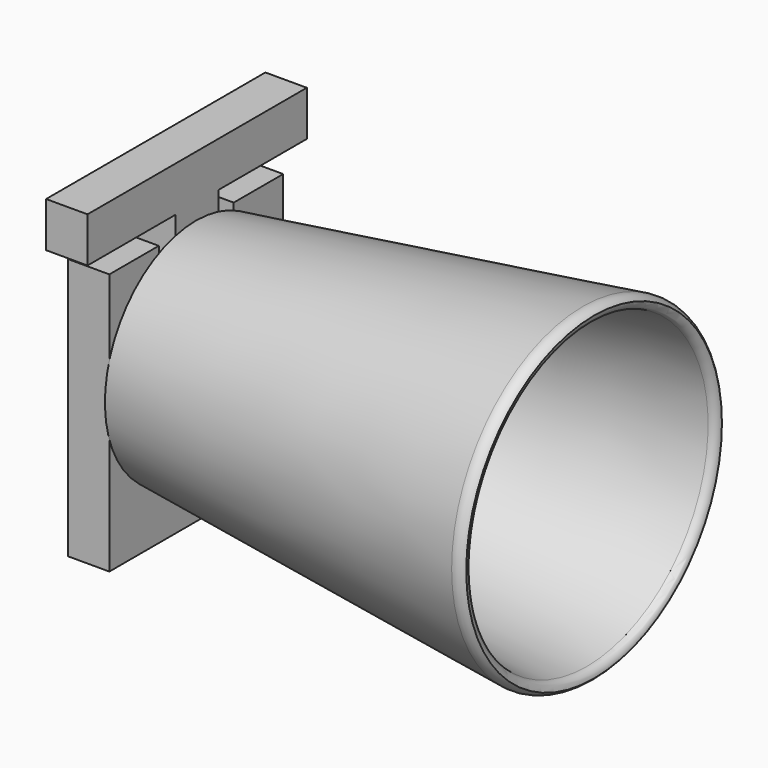
from build123d import *

# Parameters (mm, degrees)
F2_R     = 17.4625
F3_R     = 1.27
F7_DEPTH = 6.35


# Not quite as in the source:
# - a fillet or chamfer that OpenCascade refuses, or shapes differently, is made with other operations: its cross-section is extruded or revolved along the edge and cut away or added


with BuildPart() as f1:
    # F0 (on Front) → F1 (revolve)
    with BuildSketch(Plane.XZ):
        Polygon((0, 17.4625), (0, 15.4798403605), (3.3970845398, 15.9191861749), (60.9941408038, 23.3682282269), (60.9941408038, 25.4), align=None)
        Polygon((3.3970845398, 15.9191861749), (0, 15.4798403605), (0, 0), (3.3970845398, 0), align=None)
    revolve(axis=Axis((30.1625, 0, 0), (1, 0, 0)))

    # F2
    f2_edges = [f1.edges().sort_by_distance(p)[0] for p in [
        (3.397085, 0, -15.919186),
    ]]
    fillet(f2_edges, radius=F2_R)

    # F3
    f3_edges = [f1.edges().sort_by_distance(p)[0] for p in [
        (60.994141, 0, -23.368228),
    ]]
    fillet(f3_edges, radius=F3_R)

    # F4: fillet of radius 1.905 on 1 edges, made by hand

    # F4_s1 → F4_t2 (revolve, cut)
    with BuildSketch(Plane.XZ):
        with BuildLine():
            ThreePointArc((60.9944516934, 24.4848076553), (60.2207035097, 25.0552991923), (59.2669390878, 25.1756331992))
            Line((59.2669390878, 25.1756331992), (59.2423403965, 25.3646569527))
            ThreePointArc((59.2423403965, 25.3646569527), (60.1059670639, 25.4766420254), (60.9695421125, 25.5890237535))
            Line((60.9695421125, 25.5890237535), (61.1847584185, 25.4))
            ThreePointArc((61.1847584185, 25.4), (61.1847584185, 24.9424038276), (61.1426042626, 24.6047488544))
            Line((61.1426042626, 24.6047488544), (60.9944516934, 24.4848076553))
        make_face()
    revolve(axis=Axis((60.9941408038, 0, 0), (1, 0, 0)), mode=Mode.SUBTRACT)


with BuildPart() as f7:
    # F6 (on offset) → F7 (new body)
    with BuildSketch(Plane.YZ.offset(-6.35)):
        Polygon((-16.6146121919, -23.1440894544), (16.686482355, -23.1440894544), (16.686482355, 16.9517148048), (7.2066797875, 16.9517148048), (7.2066797875, -15.3657568857), (-7.1404121919, -15.3657568857), (-7.1404121919, 16.9517148048), (-16.6146121919, 16.9517148048), align=None)
    extrude(amount=F7_DEPTH)


with BuildPart() as f7b:
    # F6 (on offset) → F7, piece 2 (new body)
    with BuildSketch(Plane.YZ.offset(-6.35)):
        Polygon((21.2100986391, 26.752922684), (-20.796822384, 26.752922684), (-20.796822384, 19.8473148048), (-3.9551745407, 19.8473148048), (-4.2437847807, -12.4701568857), (4.3110797875, -12.4701568857), (4.3110797875, 19.8473148048), (21.2100986391, 19.8473148048), align=None)
    extrude(amount=F7_DEPTH)


solid = Compound([f1.part, f7.part, f7b.part])
